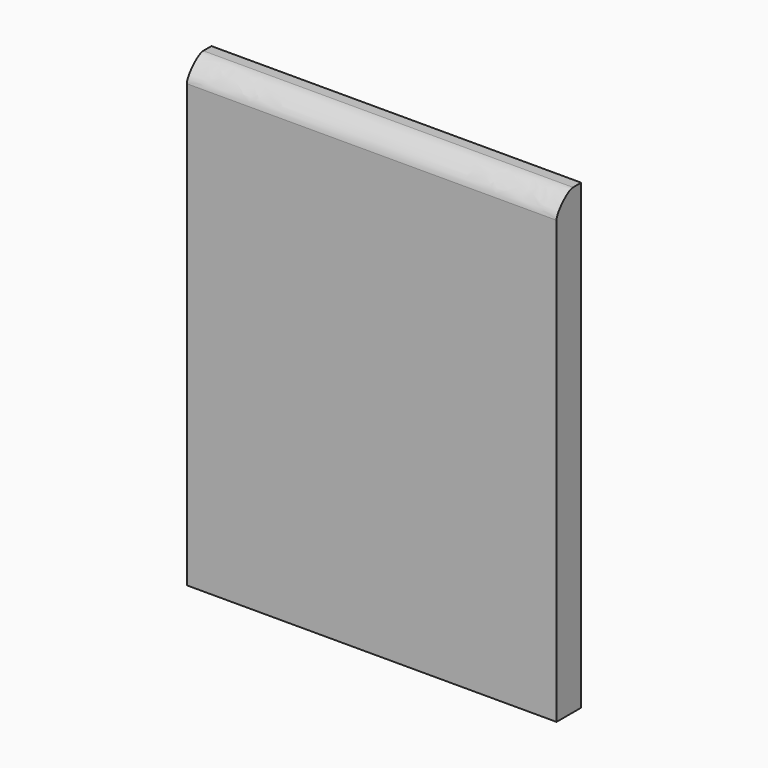
from build123d import *

# Parameters (mm, degrees)
F1_DEPTH    = 19.05
F2_T1_DEPTH = 292.1


# Not quite as in the source:
# - a fillet or chamfer that OpenCascade refuses, or shapes differently, is made with other operations: its cross-section is extruded or revolved along the edge and cut away or added
# - a feature names something its author has since deleted; it is built from what else it names


with BuildPart() as f1:
    # F0 (on Front) → F1 (new body)
    with BuildSketch(Plane.XZ):
        Polygon((-228.6, 0), (0, 0), (0, 228.6), (0, 285.75), (-228.6, 285.75), (-228.6, 228.6), align=None)
    extrude(amount=F1_DEPTH)

    # F2: fillet of radius 12.7 on 1 edges, made by hand

    # F2_s2 → F2_t1 (cut)
    with BuildSketch(Plane.YZ.offset(-260.35)):
        with BuildLine():
            add(Edge.make_bspline(
                [(-6.35, 285.75), (-19.05, 285.75), (-19.05, 273.05)],
                knots=[0, 0, 0, 1, 1, 1], degree=2, weights=[1, 0.3333333333, 1]))
            Line((-19.05, 273.05), (-19.05, 285.75))
            Line((-19.05, 285.75), (-6.35, 285.75))
        make_face()
    extrude(amount=F2_T1_DEPTH, mode=Mode.SUBTRACT)


solid = f1.part
